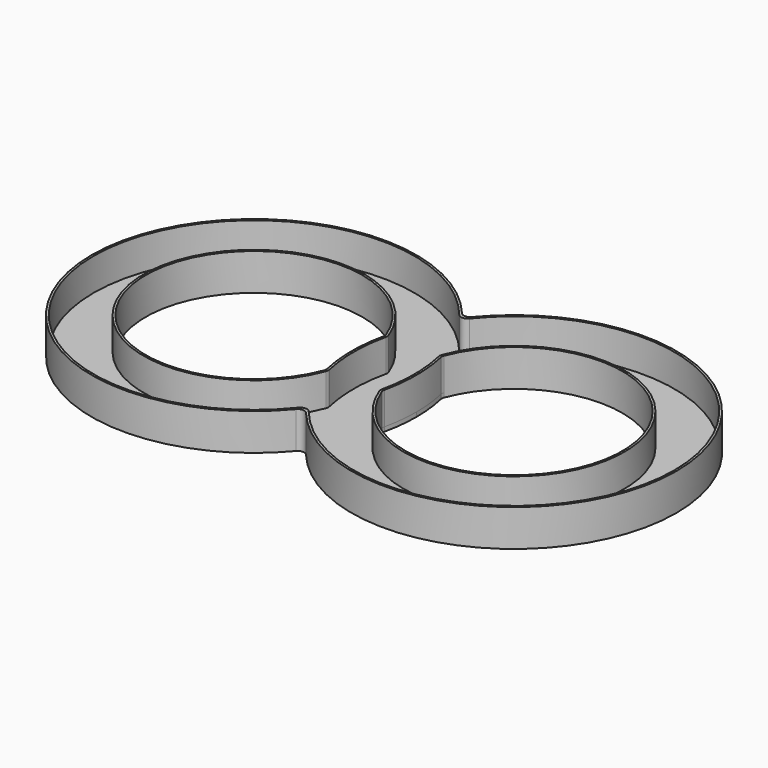
from build123d import *

# Parameters (mm, degrees)
F1_DEPTH = 2
F3_DEPTH = 15
F4_R     = 3


with BuildPart() as f1:
    # F0 (on Top) → F1 (new body)
    with BuildSketch(Plane.XY):
        with BuildLine():
            ThreePointArc((46.9791666667, 17.11601295), (49.2390004637, 8.6902723394), (50, 0))
            ThreePointArc((50, 0), (49.2390004637, -8.6902723394), (46.9791666667, -17.11601295))
            ThreePointArc((46.9791666667, -17.11601295), (52.0440237461, -31.7330315504), (60, -45))
            ThreePointArc((60, -45), (67.9559762539, -31.7330315504), (73.0208333333, -17.11601295))
            ThreePointArc((73.0208333333, -17.11601295), (70, 0), (73.0208333333, 17.11601295))
            ThreePointArc((73.0208333333, 17.11601295), (67.9559762539, 31.7330315504), (60, 45))
            ThreePointArc((60, 45), (52.0440237461, 31.7330315504), (46.9791666667, 17.11601295))
        make_face()
        with BuildLine():
            ThreePointArc((46.9791666667, -17.11601295), (-50, 0), (46.9791666667, 17.11601295))
            ThreePointArc((46.9791666667, 17.11601295), (52.0440237461, 31.7330315504), (60, 45))
            ThreePointArc((60, 45), (-75, 0), (60, -45))
            ThreePointArc((60, -45), (52.0440237461, -31.7330315504), (46.9791666667, -17.11601295))
        make_face()
        with BuildLine():
            ThreePointArc((195, 0), (143.7170824513, 71.1512473538), (60, 45))
            ThreePointArc((60, 45), (67.9559762539, 31.7330315504), (73.0208333333, 17.11601295))
            ThreePointArc((73.0208333333, 17.11601295), (128.6902723394, 49.2390004637), (170, 0))
            ThreePointArc((170, 0), (128.6902723394, -49.2390004637), (73.0208333333, -17.11601295))
            ThreePointArc((73.0208333333, -17.11601295), (67.9559762539, -31.7330315504), (60, -45))
            ThreePointArc((60, -45), (143.7170824513, -71.1512473538), (195, 0))
        make_face()
        with BuildLine():
            ThreePointArc((46.9791666667, -17.11601295), (49.2390004637, -8.6902723394), (50, 0))
            ThreePointArc((50, 0), (49.2390004637, 8.6902723394), (46.9791666667, 17.11601295))
            ThreePointArc((46.9791666667, 17.11601295), (45, 0), (46.9791666667, -17.11601295))
        make_face()
        with BuildLine():
            ThreePointArc((75, 0), (74.5035653509, 8.6150304701), (73.0208333333, 17.11601295))
            ThreePointArc((73.0208333333, 17.11601295), (70, 0), (73.0208333333, -17.11601295))
            ThreePointArc((73.0208333333, -17.11601295), (74.5035653509, -8.6150304701), (75, 0))
        make_face()
    extrude(amount=F1_DEPTH)

    # F2 (on face) → F3 (join)
    with BuildSketch(Plane.XY.offset(2)):
        with BuildLine():
            ThreePointArc((60, 45), (-75, 0), (60, -45))
            ThreePointArc((60, -45), (195, 0), (60, 45))
        make_face()
        with BuildLine():
            ThreePointArc((60, -43.3128156554), (-74, 0), (60, 43.3128156554))
            ThreePointArc((60, 43.3128156554), (194, 0), (60, -43.3128156554))
        make_face(mode=Mode.SUBTRACT)
        with BuildLine():
            ThreePointArc((48.0208333333, -17.1755514023), (46, 0), (48.0208333333, 17.1755514023))
            ThreePointArc((48.0208333333, 17.1755514023), (-51, 0), (48.0208333333, -17.1755514023))
        make_face()
        with BuildLine():
            ThreePointArc((46.9791666667, -17.11601295), (-50, 0), (46.9791666667, 17.11601295))
            ThreePointArc((46.9791666667, 17.11601295), (45, 0), (46.9791666667, -17.11601295))
        make_face(mode=Mode.SUBTRACT)
        with BuildLine():
            ThreePointArc((71.9791666667, 17.1755514023), (74, 0), (71.9791666667, -17.1755514023))
            ThreePointArc((71.9791666667, -17.1755514023), (171, 0), (71.9791666667, 17.1755514023))
        make_face()
        with BuildLine():
            ThreePointArc((73.0208333333, 17.11601295), (170, 0), (73.0208333333, -17.11601295))
            ThreePointArc((73.0208333333, -17.11601295), (75, 0), (73.0208333333, 17.11601295))
        make_face(mode=Mode.SUBTRACT)
    extrude(amount=F3_DEPTH)

    # F4
    f4_edges = [f1.edges().sort_by_distance(p)[0] for p in [
        (60, 45, 8.5),
        (60, -45, 8.5),
        (60, 43.312816, 9.5),
        (71.979167, -17.175551, 9.5),
        (73.020833, -17.116013, 8.5),
        (73.020833, 17.116013, 8.5),
        (48.020833, 17.175551, 9.5),
        (46.979167, 17.116013, 8.5),
        (46.979167, -17.116013, 8.5),
        (60, -43.312816, 9.5),
        (48.020833, -17.175551, 9.5),
        (71.979167, 17.175551, 9.5),
    ]]
    fillet(f4_edges, radius=F4_R)


solid = f1.part
